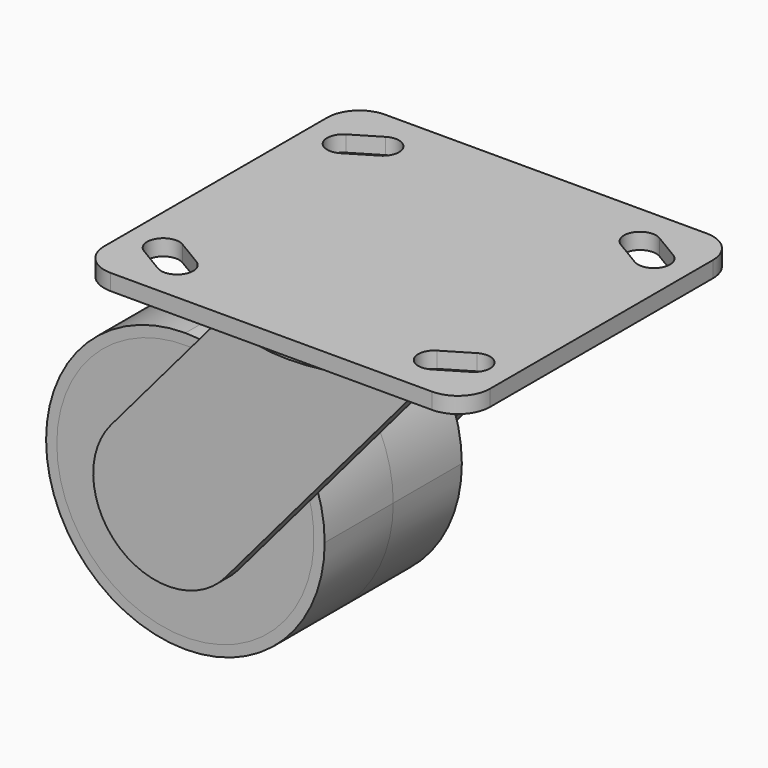
from build123d import *

# Parameters (mm, degrees)
F1_DEPTH  = 2.38125
F3_DEPTH  = 25.4
F4_R      = 44.704
F5_DEPTH  = 4.7625
F6_R      = 38.1
F7_DEPTH  = 3.175
F8_SIZE   = 3.17499
F10_DEPTH = 25.4
F12_DEPTH = 6.35
F13_DEPTH = 1.5875
F14_R     = 38.1
F15_DEPTH = 50.8
F16_DEPTH = 50.8
F18_DEPTH = 6.35
F19_DEPTH = 1.5875


# Not quite as in the source:
# - a fillet or chamfer is up to 0.001 mm smaller than in the source, because OpenCascade refuses the exact size


with BuildPart() as f1:
    # F0 (on Top) → F1 (new body, symmetric)
    with BuildSketch(Plane.XY):
        with BuildLine():
            ThreePointArc((57.15, 41.275), (54.3601920908, 48.0101920908), (47.625, 50.8))
            Line((47.625, 50.8), (-47.625, 50.8))
            ThreePointArc((-47.625, 50.8), (-54.3601920908, 48.0101920908), (-57.15, 41.275))
            Line((-57.15, 41.275), (-57.15, -41.275))
            ThreePointArc((-57.15, -41.275), (-54.3601920908, -48.0101920908), (-47.625, -50.8))
            Line((-47.625, -50.8), (47.625, -50.8))
            ThreePointArc((47.625, -50.8), (54.3601920908, -48.0101920908), (57.15, -41.275))
            Line((57.15, -41.275), (57.15, 41.275))
        make_face()
    extrude(amount=F1_DEPTH, both=True)

    # F2 (on face) → F3 (cut)
    with BuildSketch(Plane(origin=(0, 0, -2.38125), x_dir=(1, 0, 0), z_dir=(0, 0, -1))):
        with BuildLine():
            Line((-40.5502860352, 42.1838100587), (-48.4877860352, 37.4213100587))
            ThreePointArc((-48.4877860352, 37.4213100587), (-50.1213100587, 30.8872139648), (-43.5872139648, 29.2536899413))
            Line((-43.5872139648, 29.2536899413), (-35.6497139648, 34.0161899413))
            ThreePointArc((-35.6497139648, 34.0161899413), (-34.0161899413, 40.5502860352), (-40.5502860352, 42.1838100587))
        make_face()
        with BuildLine():
            Line((35.6497139648, 34.0161899413), (43.5872139648, 29.2536899413))
            ThreePointArc((43.5872139648, 29.2536899413), (50.1213100587, 30.8872139648), (48.4877860352, 37.4213100587))
            Line((48.4877860352, 37.4213100587), (40.5502860352, 42.1838100587))
            ThreePointArc((40.5502860352, 42.1838100587), (34.0161899413, 40.5502860352), (35.6497139648, 34.0161899413))
        make_face()
        with BuildLine():
            Line((-48.4877860352, -37.4213100587), (-40.5502860352, -42.1838100587))
            ThreePointArc((-40.5502860352, -42.1838100587), (-34.0161899413, -40.5502860352), (-35.6497139648, -34.0161899413))
            Line((-35.6497139648, -34.0161899413), (-43.5872139648, -29.2536899413))
            ThreePointArc((-43.5872139648, -29.2536899413), (-50.1213100587, -30.8872139648), (-48.4877860352, -37.4213100587))
        make_face()
        with BuildLine():
            Line((40.5502860352, -42.1838100587), (48.4877860352, -37.4213100587))
            ThreePointArc((48.4877860352, -37.4213100587), (50.1213100587, -30.8872139648), (43.5872139648, -29.2536899413))
            Line((43.5872139648, -29.2536899413), (35.6497139648, -34.0161899413))
            ThreePointArc((35.6497139648, -34.0161899413), (34.0161899413, -40.5502860352), (40.5502860352, -42.1838100587))
        make_face()
    extrude(amount=-F3_DEPTH, mode=Mode.SUBTRACT)

    # F4 (on face) → F5 (join)
    with BuildSketch(Plane(origin=(0, 0, -2.38125), x_dir=(1, 0, 0), z_dir=(0, 0, -1))):
        Circle(F4_R)
    extrude(amount=F5_DEPTH)


with BuildPart() as f7:
    # F6 (on face) → F7 (new body)
    with BuildSketch(Plane(origin=(0, 0, -7.14375), x_dir=(1, 0, 0), z_dir=(0, 0, -1))):
        Circle(F6_R)
    extrude(amount=F7_DEPTH)

    # F8 (size 3.175 in the source; OpenCascade refuses exactly that, so slightly less here)
    f8_edges = [f7.edges().sort_by_distance(p)[0] for p in [
        (-38.1, 0, -10.31875),
    ]]
    chamfer(f8_edges, length=F8_SIZE)


with BuildPart() as f10:
    # F9 (on Front) → F10 (new body, symmetric)
    with BuildSketch(Plane.XZ):
        with BuildLine():
            ThreePointArc((-45.8281786, -23.01875), (-75.0140109935, -35.1079176065), (-87.1031786, -64.29375))
            Line((-87.1031786, -64.29375), (-45.8281786, -64.29375))
            Line((-45.8281786, -64.29375), (-45.8281786, -23.01875))
        make_face()
        with BuildLine():
            Line((-45.8281786, -64.29375), (-87.1031786, -64.29375))
            ThreePointArc((-87.1031786, -64.29375), (-75.0140109935, -93.4795823935), (-45.8281786, -105.56875))
            Line((-45.8281786, -105.56875), (-45.8281786, -64.29375))
        make_face()
        with BuildLine():
            Line((-45.8281786, -23.01875), (-45.8281786, -64.29375))
            Line((-45.8281786, -64.29375), (-4.5531786, -64.29375))
            ThreePointArc((-4.5531786, -64.29375), (-16.6423462065, -35.1079176065), (-45.8281786, -23.01875))
        make_face()
        with BuildLine():
            Line((-4.5531786, -64.29375), (-45.8281786, -64.29375))
            Line((-45.8281786, -64.29375), (-45.8281786, -105.56875))
            ThreePointArc((-45.8281786, -105.56875), (-16.6423462065, -93.4795823935), (-4.5531786, -64.29375))
        make_face()
    extrude(amount=F10_DEPTH, both=True)

    # F14 (on face) → F15 (cut, through all)
    with BuildSketch(Plane(origin=(0, 25.4, 0), x_dir=(-1, 0, 0), z_dir=(0, 1, 0))):
        with Locations((45.8281786, -64.29375)):
            Circle(F14_R)
    extrude(amount=-F15_DEPTH, mode=Mode.SUBTRACT)


with BuildPart() as f12:
    # F11 (on face) → F12 (new body)
    with BuildSketch(Plane.XZ.offset(25.4)):
        with BuildLine():
            Line((29.1555075522, -10.31875), (-29.1555075522, -10.31875))
            Line((-29.1555075522, -10.31875), (-62.7701105528, -49.9089814337))
            ThreePointArc((-62.7701105528, -49.9089814337), (-60.2129471663, -81.2356819528), (-28.8862466472, -78.6785185663))
            Line((-28.8862466472, -78.6785185663), (16.9419319528, -24.7035185663))
            Line((16.9419319528, -24.7035185663), (29.1555075522, -10.31875))
        make_face()
    extrude(amount=F12_DEPTH)

    # F13 (cut): a face of the model
    f13_faces = [f12.faces().sort_by_distance(p)[0] for p in [
        (-27.0105853212, -25.4, -44.578171556),
    ]]
    extrude(f13_faces, amount=-F13_DEPTH, mode=Mode.SUBTRACT)


with BuildPart() as f16:
    # F14 (on face) → F16 (new body)
    with BuildSketch(Plane(origin=(0, 25.4, 0), x_dir=(-1, 0, 0), z_dir=(0, 1, 0))):
        with Locations((45.8281786, -64.29375)):
            Circle(F14_R)
    extrude(amount=-F16_DEPTH)


with BuildPart() as f18:
    # F17 (on face) → F18 (new body)
    with BuildSketch(Plane(origin=(0, 25.4, 0), x_dir=(-1, 0, 0), z_dir=(0, 1, 0))):
        with BuildLine():
            Line((62.7701105528, -49.9089814337), (42.7407704224, -26.3190490697))
            ThreePointArc((42.7407704224, -26.3190490697), (21.1685753435, -35.2504380808), (8.8569065167, -55.0885862022))
            Line((8.8569065167, -55.0885862022), (28.8862466472, -78.6785185663))
            ThreePointArc((28.8862466472, -78.6785185663), (60.2129471663, -81.2356819528), (62.7701105528, -49.9089814337))
        make_face()
        with BuildLine():
            Line((29.1555075522, -10.31875), (-29.1555075522, -10.31875))
            Line((-29.1555075522, -10.31875), (-16.9419319528, -24.7035185663))
            Line((-16.9419319528, -24.7035185663), (8.8569065167, -55.0885862022))
            ThreePointArc((8.8569065167, -55.0885862022), (21.1685753435, -35.2504380808), (42.7407704224, -26.3190490697))
            Line((42.7407704224, -26.3190490697), (29.1555075522, -10.31875))
        make_face()
    extrude(amount=F18_DEPTH)

    # F19 (cut): a face of the model
    f19_faces = [f18.faces().sort_by_distance(p)[0] for p in [
        (-27.0105853212, 25.4, -44.578171556),
    ]]
    extrude(f19_faces, amount=-F19_DEPTH, mode=Mode.SUBTRACT)


solid = Compound([f1.part, f7.part, f10.part, f12.part, f16.part, f18.part])
